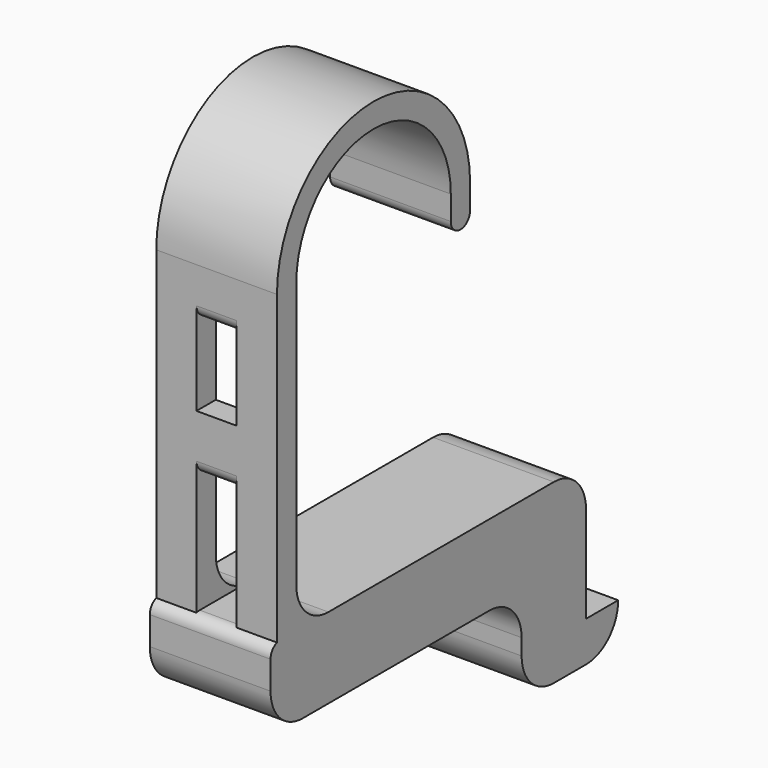
from build123d import *

# Parameters (mm, degrees)
F0_W          = 1
F0_H          = 10
F1_DEPTH      = 7.5
F1_DEPTH_BACK = 7.5
F2_W          = 5
F2_H          = 10
F2_H_2        = 15
F3_DEPTH      = 3
F4_R          = 1.49999
F5_R          = 4.99999


# Not quite as in the source:
# - a fillet or chamfer is up to 0.001 mm smaller than in the source, because OpenCascade refuses the exact size


with BuildPart() as f1:
    # F0 (on Right) → F1 (new body, two sides)
    with BuildSketch(Plane.YZ) as f1_sk:
        with BuildLine():
            ThreePointArc((-12, 0), (0, 12), (12, 0))
            Line((12, 0), (12, -3))
            ThreePointArc((12, -3), (13.5, -4.5), (15, -3))
            Line((15, -3), (15, 0))
            ThreePointArc((15, 0), (0, 15), (-15, 0))
            Line((-15, 0), (-15, -38))
            Line((-15, -38), (-15, -48))
            Line((-15, -48), (-12, -48))
            Line((-12, -48), (23, -48))
            Line((23, -48), (23, -60))
            Line((23, -60), (33, -60))
            Line((33, -60), (38, -60))
            Line((38, -60), (38, -55))
            Line((38, -55), (33, -55))
            Line((33, -55), (33, -48))
            Line((33, -48), (33, -38))
            Line((33, -38), (-12, -38))
            Line((-12, -38), (-12, 0))
        make_face()
        with Locations((-15.5, -43)):
            Rectangle(F0_W, F0_H)
    extrude(amount=F1_DEPTH)
    extrude(f1_sk.sketch, amount=-F1_DEPTH_BACK)

    # F2 (on face) → F3 (cut, through all)
    with BuildSketch(Plane.XZ.offset(15)):
        with Locations((0, -11)):
            Rectangle(F2_W, F2_H)
        with Locations((0, -30.5)):
            Rectangle(F2_W, F2_H_2)
    extrude(amount=-F3_DEPTH, mode=Mode.SUBTRACT)

    # F4 (radius 1.5 in the source; OpenCascade refuses exactly that, so slightly less here)
    f4_edges = [f1.edges().sort_by_distance(p)[0] for p in [
        (0, -15, -6),
        (0, -12, -6),
        (0, -15, -23),
        (0, -12, -23),
        (0, -16, -38),
    ]]
    fillet(f4_edges, radius=F4_R)

    # F5 (radius 5 in the source; OpenCascade refuses exactly that, so slightly less here)
    f5_edges = [f1.edges().sort_by_distance(p)[0] for p in [
        (5, -12, -38),
        (-5, -12, -38),
        (0, 33, -38),
        (0, 38, -60),
        (0, 23, -60),
        (0, 23, -48),
        (0, -15, 0),
        (0, -16, -48),
    ]]
    fillet(f5_edges, radius=F5_R)


solid = f1.part
